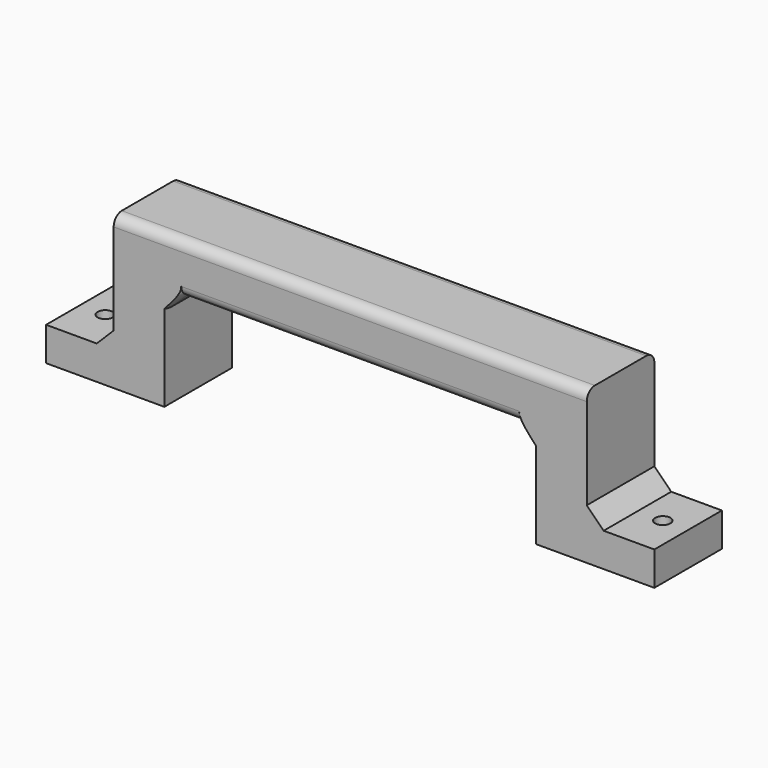
from build123d import *

# Parameters (mm, degrees)
F1_DEPTH     = 25
F2_R         = 3
F3_T1_DEPTH  = 25
F3_T3_DEPTH  = 19
F3_T8_ANGLE  = 335.676286299
F3_T13_ANGLE = 335.676286299
F3_T18_ANGLE = 335.676286299
F3_T23_ANGLE = 335.676286299
F4_R         = 2.25
F5_DEPTH     = 10.001
F6_TEXT_SIZE = 13.1947891159
F7_DEPTH     = 3


# Not quite as in the source:
# - a fillet or chamfer that OpenCascade refuses, or shapes differently, is made with other operations: its cross-section is extruded or revolved along the edge and cut away or added
# - Text() gives the source's letters only with a copy of the font that has no kerning and outlines rounded to 1/6400 em; it was checked with that copy


with BuildPart() as f1:
    # F0 (on Front) → F1 (new body)
    with BuildSketch(Plane.XZ):
        Polygon((0, 10), (0, 0), (35, 0), (35, 30), (90, 30), (145, 30), (145, 0), (180, 0), (180, 10), (160, 10), (160, 45), (90, 45), (20, 45), (20, 10), align=None)
    extrude(amount=F1_DEPTH)

    # F2
    f2_edges = [f1.edges().sort_by_distance(p)[0] for p in [
        (90, -25, 45),
        (90, 0, 45),
        (90, -25, 30),
        (90, 0, 30),
    ]]
    fillet(f2_edges, radius=F2_R)

    # F3: chamfer of 5 on 4 edges, made by hand

    # F3_s2 → F3_t1 (join)
    with BuildSketch(Plane.XZ):
        Polygon((20, 15), (15, 10), (20, 10), align=None)
        Polygon((160, 15), (165, 10), (160, 10), align=None)
    extrude(amount=F3_T1_DEPTH)

    # F3_s4 → F3_t3 (join)
    with BuildSketch(Plane.XZ.offset(3)):
        Polygon((35, 25), (40, 30), (35, 30), align=None)
        Polygon((145, 25), (140, 30), (145, 30), align=None)
    extrude(amount=F3_T3_DEPTH)


with BuildPart() as f3_tool6:
    # F3_s7 → F3_t8 (revolve)
    with BuildSketch(Plane.XZ.offset(3)):
        Polygon((145, 25), (140, 30), (145, 30), align=None)
    revolve(axis=Axis((145, -3, 33), (1, 0, 0)), revolution_arc=F3_T8_ANGLE)

    split(bisect_by=Plane.XZ, keep=Keep.TOP)


with BuildPart() as f1_1:
    add(f1.part)

    # F3_t5: union F3_tool6
    add(f3_tool6.part)


with BuildPart() as f3_tool11:
    # F3_s12 → F3_t13 (revolve)
    with BuildSketch(Plane(origin=(0, -5.8817372815, -2.6586373927), x_dir=(1, 0, 0), z_dir=(0, -0.9112328801, -0.4118915369))):
        Polygon((145, 31.1322988561), (140, 36.1322988561), (145, 36.1322988561), align=None)
    revolve(axis=Axis((145, -22, 33), (1, 0, 0)), revolution_arc=F3_T13_ANGLE)

    split(bisect_by=Plane.XZ.offset(25), keep=Keep.BOTTOM)


with BuildPart() as f1_2:
    add(f1_1.part)

    # F3_t10: union F3_tool11
    add(f3_tool11.part)


with BuildPart() as f3_tool16:
    # F3_s17 → F3_t18 (revolve)
    with BuildSketch(Plane.XZ.offset(3)):
        Polygon((35, 25), (40, 30), (35, 30), align=None)
    revolve(axis=Axis((35, -3, 33), (1, 0, 0)), revolution_arc=F3_T18_ANGLE)

    split(bisect_by=Plane.XZ, keep=Keep.TOP)


with BuildPart() as f1_3:
    add(f1_2.part)

    # F3_t15: union F3_tool16
    add(f3_tool16.part)


with BuildPart() as f3_tool21:
    # F3_s22 → F3_t23 (revolve)
    with BuildSketch(Plane(origin=(0, -5.8817372815, -2.6586373927), x_dir=(1, 0, 0), z_dir=(0, -0.9112328801, -0.4118915369))):
        Polygon((35, 31.1322988561), (40, 36.1322988561), (35, 36.1322988561), align=None)
    revolve(axis=Axis((35, -22, 33), (1, 0, 0)), revolution_arc=F3_T23_ANGLE)

    split(bisect_by=Plane.XZ.offset(25), keep=Keep.BOTTOM)


with BuildPart() as f1_4:
    add(f1_3.part)

    # F3_t20: union F3_tool21
    add(f3_tool21.part)

    # F4 (on face) → F5 (cut, through all)
    with BuildSketch(Plane.XY.offset(10)):
        with Locations((7.5, -12.5)):
            Circle(F4_R)
        with Locations((172.5, -12.5)):
            Circle(F4_R)
    extrude(amount=-F5_DEPTH, mode=Mode.SUBTRACT)

    # F6 (on face) → F7 (cut)
    with BuildSketch(Plane(origin=(0, 0, 30), x_dir=(1, 0, 0), z_dir=(0, 0, -1))):
        with Locations((76.2650492046, 9.0113235638)):
            Text('RMF', F6_TEXT_SIZE, font='Open Sans', text_align=(TextAlign.LEFT, TextAlign.BOTTOM))
    extrude(amount=-F7_DEPTH, mode=Mode.SUBTRACT)


solid = f1_4.part
